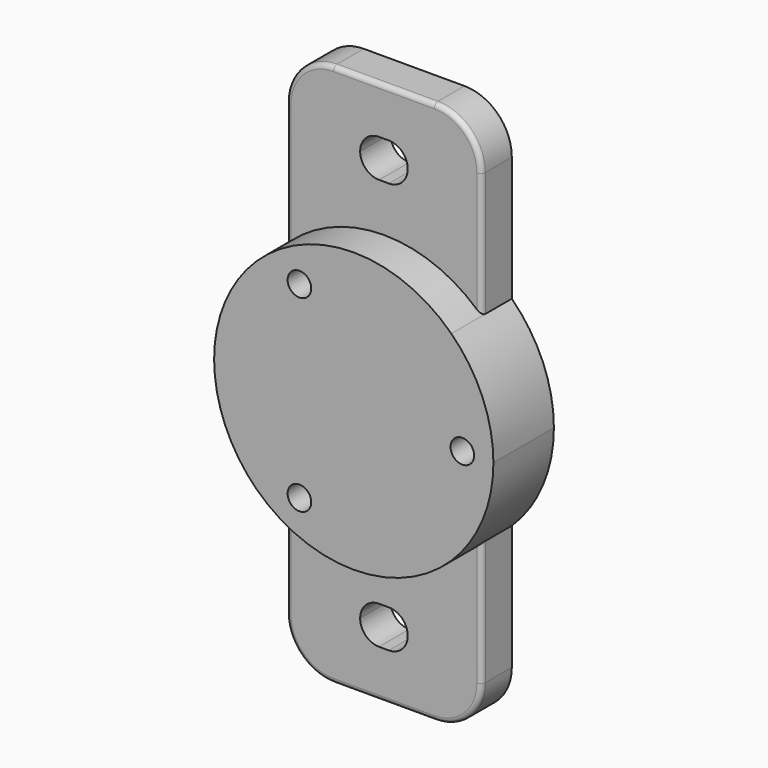
from build123d import *

# Parameters (mm, degrees)
F0_W          = 41.3257516921
F0_H          = 115.0570958853
F1_DEPTH      = 8
F3_DEPTH      = 16
F5_DEPTH      = 8.5
F6_R          = 4
F7_R          = 10
F9_D          = 5
F10_R         = 1
F12_DEPTH     = 8
F13_T4_ANGLE  = 50.4345634546
F13_S5_R      = 29.5691559209
F13_T6_DEPTH  = 16
F13_T11_ANGLE = 49.9258142249
F13_S12_R     = 29.5691559209
F13_T13_DEPTH = 16
F14_W         = 7.5
F14_H         = 18
F15_DEPTH     = 3
F16_R         = 1


# Not quite as in the source:
# - a fillet or chamfer that OpenCascade refuses, or shapes differently, is made with other operations: its cross-section is extruded or revolved along the edge and cut away or added
# - a pattern or mirror of a feature is missing from the dataset's text; its kind, count and spacing are read off the source's solid


with BuildPart() as f1:
    # F0 (on Front) → F1 (new body)
    with BuildSketch(Plane.XZ):
        Rectangle(F0_W, F0_H)
    extrude(amount=F1_DEPTH)

    # F2 (on face) → F3 (join)
    with BuildSketch(Plane.XZ):
        with BuildLine():
            Line((20.662875846, -21.1513721457), (20.662875846, 21.1513721457))
            ThreePointArc((20.662875846, 21.1513721457), (0, 29.5691559209), (-20.662875846, 21.1513721457))
            Line((-20.662875846, 21.1513721457), (-20.662875846, -21.1513721457))
            ThreePointArc((-20.662875846, -21.1513721457), (0, -29.5691559209), (20.662875846, -21.1513721457))
        make_face()
        with BuildLine():
            ThreePointArc((20.662875846, -21.1513721457), (27.251777736, -11.4749985666), (29.5691559209, 0))
            ThreePointArc((29.5691559209, 0), (27.251777736, 11.4749985666), (20.662875846, 21.1513721457))
            Line((20.662875846, 21.1513721457), (20.662875846, -21.1513721457))
        make_face()
    extrude(amount=F3_DEPTH)

    # F4 (on face) → F5 (cut)
    with BuildSketch(Plane(origin=(0, 0, 0), x_dir=(-1, 0, 0), z_dir=(0, 1, 0))):
        Polygon((5.0357980654, 39.4895523787), (5.0357980654, 47.5048683584), (-5.0371875986, 47.5048683584), (-5.0371875986, 39.4847430289), align=None)
    f5 = extrude(amount=-F5_DEPTH, mode=Mode.SUBTRACT)

    # F5_copies: F5 across plane
    add(f5.mirror(Plane(origin=(0, 0, 0), x_dir=(-1, 0, 0), z_dir=(0, 0, -1))), mode=Mode.SUBTRACT)

    # F6
    f6_edges = [f1.edges().sort_by_distance(p)[0] for p in [
        (5.037188, -4, -47.504868),
        (-5.035798, -4, -47.504868),
        (5.037188, -4, -39.484743),
        (-5.035798, -4, -39.489552),
        (-5.035798, -4, 47.504868),
        (-5.035798, -4, 39.489552),
        (5.037188, -4, 39.484743),
        (5.037188, -4, 47.504868),
    ]]
    fillet(f6_edges, radius=F6_R)

    # F7
    f7_edges = [f1.edges().sort_by_distance(p)[0] for p in [
        (20.662876, -4, 57.528548),
        (-20.662876, -4, 57.528548),
        (-20.662876, -4, -57.528548),
        (20.662876, -4, -57.528548),
    ]]
    fillet(f7_edges, radius=F7_R)

    # F8: union 

    # F9 (through all)
    with Locations(Plane(origin=(0, 0, 0), x_dir=(1, 0, 0), z_dir=(0, 1, 0))):
        with Locations((22.990738973, 0), (-11.4866392687, -19.9111644179), (-11.4866392687, 19.9130717665)):
            Hole(F9_D / 2)

    # F10
    f10_edges = [f1.edges().sort_by_distance(p)[0] for p in [
        (-20.662876, -8, 34.33996),
        (-20.662876, -8, -34.33996),
    ]]
    fillet(f10_edges, radius=F10_R)

    # F11 (on face) → F12 (join)
    with BuildSketch(Plane.XZ.offset(16)):
        with BuildLine():
            ThreePointArc((-20.662875846, 21.1513721457), (-27.2355425635, 11.47094423), (-29.5438040048, 0))
            ThreePointArc((-29.5438040048, 0), (-27.2133537023, -11.4616276864), (-20.662875846, -21.1513721457))
            Line((-20.662875846, -21.1513721457), (-20.662875846, 21.1513721457))
        make_face()
    extrude(amount=-F12_DEPTH)

    # F13: fillet of radius 1 on 2 edges, made by hand


with BuildPart() as f13_tool2:
    # F13_s3 → F13_t4 (revolve)
    with BuildSketch(Plane(origin=(0.039948819, 0, 0.0330329638), x_dir=(0, 1, 0), z_dir=(0.7706607763, 0, 0.6372456103))):
        with BuildLine():
            ThreePointArc((-9, 29.573386115), (-8.2928932188, 29.2804928962), (-8, 28.573386115))
            Line((-8, 28.573386115), (-7.98, 28.573386115))
            Line((-7.98, 28.573386115), (-7.98, 29.593386115))
            Line((-7.98, 29.593386115), (-9, 29.593386115))
            Line((-9, 29.593386115), (-9, 29.573386115))
        make_face()
    revolve(axis=Axis((0.058163466, -8, 0.0110048576), (0, -1, 0)), revolution_arc=F13_T4_ANGLE)

    # F13_s5 → F13_t6 (intersect, symmetric)
    with BuildSketch(Plane.XZ.offset(8.5)):
        Circle(F13_S5_R)
    extrude(amount=F13_T6_DEPTH, both=True, mode=Mode.INTERSECT)

    split(bisect_by=Plane.YZ.offset(-20.662875846), keep=Keep.BOTTOM)


with BuildPart() as f1_1:
    add(f1.part)

    # F13_t1: cut F13_tool2
    add(f13_tool2.part, mode=Mode.SUBTRACT)


with BuildPart() as f13_tool9:
    # F13_s10 → F13_t11 (revolve)
    with BuildSketch(Plane(origin=(-0.0003962248, 0, 0.1081934909), x_dir=(0, 1, 0), z_dir=(-0.0036621627, 0, 0.9999932943))):
        with BuildLine():
            ThreePointArc((-9, 29.5436058917), (-8.2928932188, 29.2507126729), (-8, 28.5436058917))
            Line((-8, 28.5436058917), (-7.98, 28.5436058917))
            Line((-7.98, 28.5436058917), (-7.98, 29.5636058917))
            Line((-7.98, 29.5636058917), (-9, 29.5636058917))
            Line((-9, 29.5636058917), (-9, 29.5436058917))
        make_face()
    revolve(axis=Axis((0.3450668448, -8, 0.1094586414), (0, -1, 0)), revolution_arc=F13_T11_ANGLE)

    # F13_s12 → F13_t13 (intersect, symmetric)
    with BuildSketch(Plane.XZ.offset(8.5)):
        Circle(F13_S12_R)
    extrude(amount=F13_T13_DEPTH, both=True, mode=Mode.INTERSECT)

    split(bisect_by=Plane.YZ.offset(-20.662875846), keep=Keep.BOTTOM)


with BuildPart() as f1_2:
    add(f1_1.part)

    # F13_t8: cut F13_tool9
    add(f13_tool9.part, mode=Mode.SUBTRACT)

    # F14 (on face) → F15 (join)
    with BuildSketch(Plane(origin=(0, 0, 0), x_dir=(-1, 0, 0), z_dir=(0, 1, 0))):
        with Locations((0, -21)):
            Rectangle(F14_W, F14_H)
        with Locations((0, 21)):
            Rectangle(F14_W, F14_H)
    extrude(amount=F15_DEPTH)

    # F16
    f16_edges = [f1_2.edges().sort_by_distance(p)[0] for p in [
        (3.75, 3, 21),
        (0, 3, 12),
        (-3.75, 3, 21),
        (0, 3, 30),
        (0, 3, -12),
        (3.75, 3, -21),
        (0, 3, -30),
        (-3.75, 3, -21),
    ]]
    fillet(f16_edges, radius=F16_R)


solid = f1_2.part
